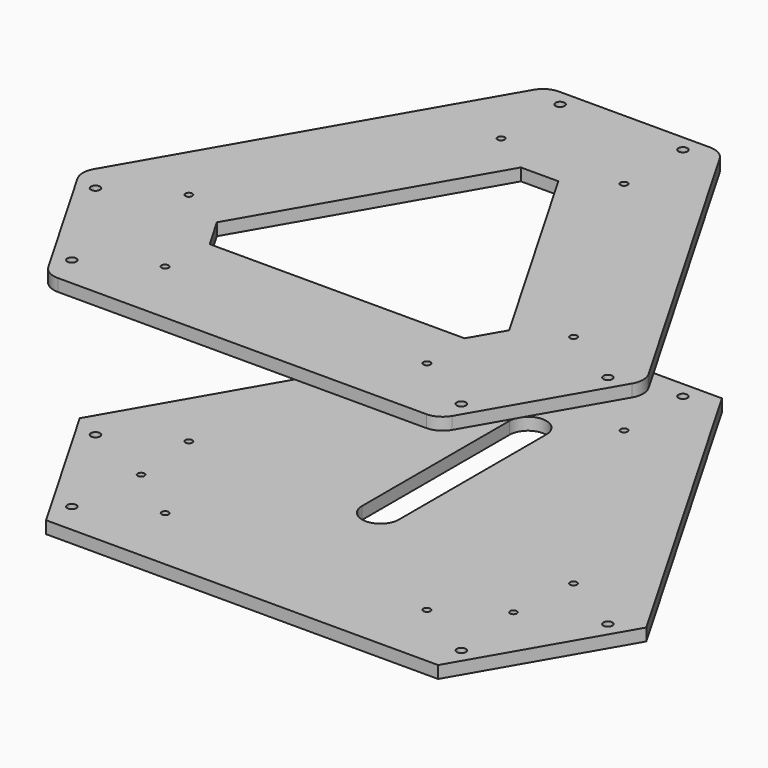
from build123d import *

# Parameters (mm, degrees)
F0_R     = 2.2
F0_R_2   = 1.7
F1_DEPTH = 6
F3_R     = 2.2
F3_R_2   = 1.7
F3_R_3   = 1.65
F4_DEPTH = 6
F5_R     = 10


# Not quite as in the source:
# - a feature names something its author has since deleted; it is built from what else it names


with BuildPart() as f1:
    # F0 (on Top) → F1 (new body)
    with BuildSketch(Plane.XY):
        Polygon((-42.617, 135.14210956), (-138.345, -30.6636501469), (-95.728, -104.4784594131), (95.728, -104.4784594131), (138.345, -30.6636501469), (42.617, 135.14210956), align=None)
        with Locations((-95.1082967697, -89.5518168935)):
            Circle(F0_R, mode=Mode.SUBTRACT)
        with Locations((-63.9313822335, -71.5518168935)):
            Circle(F0_R_2, mode=Mode.SUBTRACT)
        with Locations((-125.1082967697, -37.5902926665)):
            Circle(F0_R, mode=Mode.SUBTRACT)
        with Locations((-93.9313822335, -19.5902926665)):
            Circle(F0_R_2, mode=Mode.SUBTRACT)
        Polygon((71.372368774, -30.6636501469), (62.241684387, -46.4784594131), (-62.241684387, -46.4784594131), (-71.372368774, -30.6636501469), (-9.130684387, 77.14210956), (9.130684387, 77.14210956), align=None, mode=Mode.SUBTRACT)
        with Locations((63.9313822335, -71.5518168935)):
            Circle(F0_R_2, mode=Mode.SUBTRACT)
        with Locations((95.1082967697, -89.5518168935)):
            Circle(F0_R, mode=Mode.SUBTRACT)
        with Locations((93.9313822335, -19.5902926665)):
            Circle(F0_R_2, mode=Mode.SUBTRACT)
        with Locations((125.1082967697, -37.5902926665)):
            Circle(F0_R, mode=Mode.SUBTRACT)
        with Locations((-30, 91.14210956)):
            Circle(F0_R_2, mode=Mode.SUBTRACT)
        with Locations((-30, 127.14210956)):
            Circle(F0_R, mode=Mode.SUBTRACT)
        with Locations((30, 91.14210956)):
            Circle(F0_R_2, mode=Mode.SUBTRACT)
        with Locations((30, 127.14210956)):
            Circle(F0_R, mode=Mode.SUBTRACT)
    extrude(amount=F1_DEPTH)

    # F5
    f5_edges = [f1.edges().sort_by_distance(p)[0] for p in [
        (95.728, -104.478459, 3),
        (138.345, -30.66365, 3),
        (-95.728, -104.478459, 3),
        (-138.345, -30.66365, 3),
        (-42.617, 135.14211, 3),
        (42.617, 135.14211, 3),
    ]]
    fillet(f5_edges, radius=F5_R)


with BuildPart() as f4:
    # F3 (on offset) → F4 (new body)
    with BuildSketch(Plane(origin=(0, 0, -100), x_dir=(1, 0, 0), z_dir=(0, 0, -1))):
        Polygon((95.728, 104.4784594131), (-95.728, 104.4784594131), (-138.345, 30.6636501469), (-42.617, -135.14210956), (42.617, -135.14210956), (138.345, 30.6636501469), align=None)
        with Locations((-30, -127.14210956)):
            Circle(F3_R, mode=Mode.SUBTRACT)
        with Locations((-30, -91.14210956)):
            Circle(F3_R_2, mode=Mode.SUBTRACT)
        with Locations((0, -105)):
            Circle(F3_R_3, mode=Mode.SUBTRACT)
        with BuildLine():
            Line((-9, -70), (-9, 20))
            ThreePointArc((-9, 20), (0, 29), (9, 20))
            Line((9, 20), (9, -70))
            ThreePointArc((9, -70), (0, -79), (-9, -70))
        make_face(mode=Mode.SUBTRACT)
        with Locations((30, -127.14210956)):
            Circle(F3_R, mode=Mode.SUBTRACT)
        with Locations((30, -91.14210956)):
            Circle(F3_R_2, mode=Mode.SUBTRACT)
        with Locations((-125.1082967697, 37.5902926665)):
            Circle(F3_R, mode=Mode.SUBTRACT)
        with Locations((-93.9313822335, 19.5902926665)):
            Circle(F3_R_2, mode=Mode.SUBTRACT)
        with Locations((-90.9326673974, 52.5)):
            Circle(F3_R_3, mode=Mode.SUBTRACT)
        with Locations((-95.1082967697, 89.5518168935)):
            Circle(F3_R, mode=Mode.SUBTRACT)
        with Locations((-63.9313822335, 71.5518168935)):
            Circle(F3_R_2, mode=Mode.SUBTRACT)
        with Locations((93.9313822335, 19.5902926665)):
            Circle(F3_R_2, mode=Mode.SUBTRACT)
        with Locations((125.1082967697, 37.5902926665)):
            Circle(F3_R, mode=Mode.SUBTRACT)
        with Locations((63.9313822335, 71.5518168935)):
            Circle(F3_R_2, mode=Mode.SUBTRACT)
        with Locations((90.9326673974, 52.5)):
            Circle(F3_R_3, mode=Mode.SUBTRACT)
        with Locations((95.1082967697, 89.5518168935)):
            Circle(F3_R, mode=Mode.SUBTRACT)
    extrude(amount=F4_DEPTH)


solid = Compound([f1.part, f4.part])
